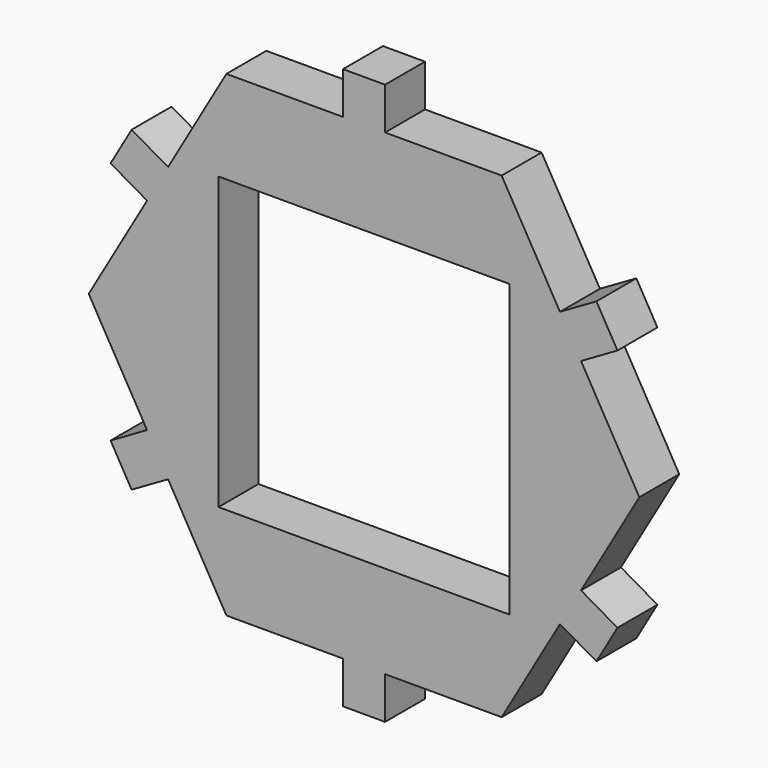
from build123d import *

# Parameters (mm, degrees)
F1_DEPTH = 6.35
F2_W     = 5.35
F2_H     = 5.35
F3_DEPTH = 6.35
F4_W     = 37
F4_H     = 37
F5_DEPTH = 25


# Not quite as in the source:
# - a length typed as a fraction of an inch, garbled in the dataset ("3 / 203.2 mm" for 3/8 in), is restored


with BuildPart() as f1:
    # F0 (on Front) → F1 (new body)
    with BuildSketch(Plane.XZ):
        Polygon((17.5, -30.3108891325), (35, 0), (17.5, 30.3108891325), (-17.5, 30.3108891325), (-35, 0), (-17.5, -30.3108891325), align=None)
    extrude(amount=F1_DEPTH)

    # F2 (on face) → F3 (join)
    with BuildSketch(Plane.XZ.offset(6.35)):
        with Locations((0, 32.9858891325)):
            Rectangle(F2_W, F2_H)
        with Locations((0, -32.9858891325)):
            Rectangle(F2_W, F2_H)
        Polygon((29.5457359102, 20.1470625214), (24.9125, 17.4720625214), (27.5875, 12.8388266111), (32.2207359102, 15.5138266111), align=None)
        Polygon((-32.2207359102, 15.5138266111), (-27.5875, 12.8388266111), (-24.9125, 17.4720625214), (-29.5457359102, 20.1470625214), align=None)
        Polygon((-24.9125, -17.4720625214), (-27.5875, -12.8388266111), (-32.2207359102, -15.5138266111), (-29.5457359102, -20.1470625214), align=None)
        Polygon((27.5875, -12.8388266111), (24.9125, -17.4720625214), (29.5457359102, -20.1470625214), (32.2207359102, -15.5138266111), align=None)
    extrude(amount=-F3_DEPTH)

    # F4 (on face) → F5 (cut)
    with BuildSketch(Plane.XZ.offset(6.35)):
        Rectangle(F4_W, F4_H)
    extrude(amount=-F5_DEPTH, mode=Mode.SUBTRACT)


solid = f1.part
